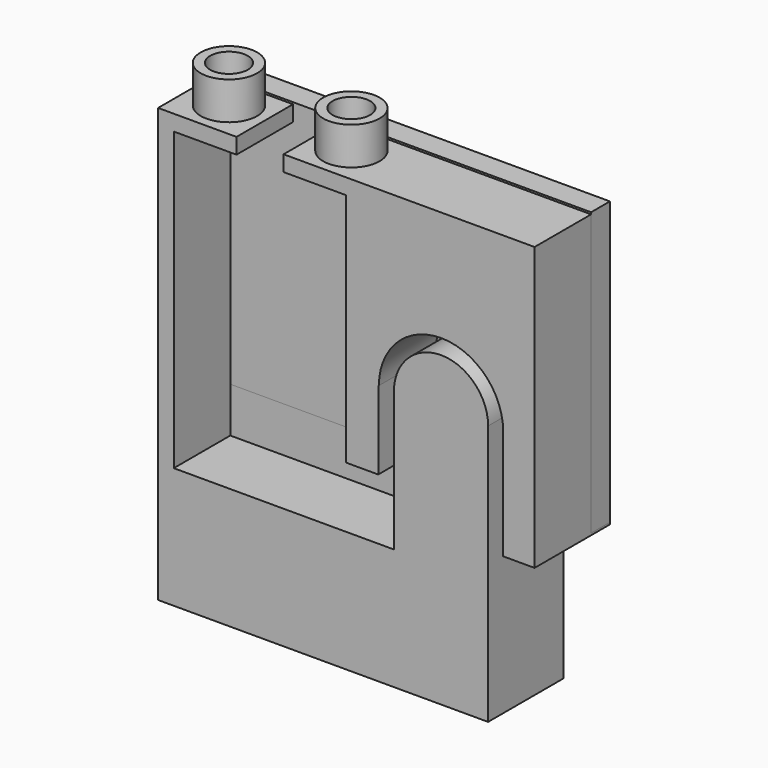
from build123d import *

# Parameters (mm, degrees)
F1_DEPTH  = 15.875
F0_W      = 2.6458333332
F0_H      = 42.3358732487
F2_W      = 63.5
F2_H      = 47.625
F2_R      = 3.175
F3_DEPTH  = 3.96875
F4_DEPTH  = 6.35
F5_R      = 4.7625
F5_R_2    = 3.175
F6_DEPTH  = 6.35
F7_R      = 3.175
F8_DEPTH  = 25.4
F9_W      = 55.6354932006
F9_H      = 15.875
F10_DEPTH = 25.4
F11_W     = 37.1146598675
F11_H     = 15.875
F12_DEPTH = 7.62
F13_W     = 37.1146598675
F13_H     = 3.96875
F14_DEPTH = 25.4


# Not quite as in the source:
# - a feature names something its author has since deleted; it is built from what else it names


with BuildPart() as f1:
    # F0 (on Front) → F1 (new body)
    with BuildSketch(Plane.XZ):
        with BuildLine():
            Line((0, 44.979166582), (-31.75, 44.979166582))
            Line((-31.75, 44.979166582), (-31.75, 42.3358732487))
            Line((-31.75, 42.3358732487), (-31.75, 2.6458333332))
            Line((-31.75, 2.6458333332), (-26.3525, 2.6458333332))
            Line((-26.3525, 2.6458333332), (-26.3525, 15.875))
            Line((-26.3525, 15.875), (-26.2466666667, 15.875))
            ThreePointArc((-26.2466666667, 15.875), (-15.7691666667, 26.3525), (-5.2916666667, 15.875))
            Line((-5.2916666667, 15.875), (-5.2916666667, 0))
            Line((-5.2916666667, 0), (0, 0))
            Line((0, 0), (0, 44.979166582))
        make_face()
        Polygon((0, -2.6458333333), (0, 0), (-5.2916666667, 0), (-5.309548229, 0), (-5.309548229, -2.6458333333), align=None)
        Polygon((-31.75, 42.3358732487), (-31.75, 44.979166582), (-34.3958333316, 44.979166582), (-37.0416664956, 44.979166582), (-42.3110765377, 44.979166582), (-42.3110765377, 42.3358732487), (-37.0416664956, 42.3358732487), (-34.3958333316, 42.3358732487), align=None)
    extrude(amount=F1_DEPTH)


with BuildPart() as f1b:
    # F0 (on Front) → F1, piece 2 (new body)
    with BuildSketch(Plane.XZ):
        with BuildLine():
            Line((-23.7066666667, 0), (-7.8316666667, 0))
            Line((-7.8316666667, 0), (-7.8316666667, 15.875))
            ThreePointArc((-7.8316666667, 15.875), (-15.7691666667, 23.8125), (-23.7066666667, 15.875))
            Line((-23.7066666667, 15.875), (-23.7066666667, 0))
        make_face()
        Polygon((-26.3525, 0), (-31.75, 0), (-60.8213265341, 0), (-63.4671598673, 0), (-63.4671598673, -2.6458333333), (-7.8316666667, -2.6458333333), (-7.8316666667, 0), (-23.7066666667, 0), align=None)
        with Locations((-62.1442432007, 21.1679366243)):
            Rectangle(F0_W, F0_H)
        Polygon((-50.2485765377, 42.3358732487), (-50.2485765377, 44.979166582), (-55.5296598693, 44.979166582), (-58.175493201, 44.979166582), (-63.4671598673, 44.979166582), (-63.4671598673, 42.3358732487), (-60.8213265341, 42.3358732487), (-58.175493201, 42.3358732487), (-55.5296598693, 42.3358732487), align=None)
    extrude(amount=F1_DEPTH)


with BuildPart() as f3:
    # F2 (on Front) → F3 (new body)
    with BuildSketch(Plane.XZ):
        with Locations((-31.75, 21.4839725468)):
            Rectangle(F2_W, F2_H)
        with Locations((-53.975, 7.1964725468)):
            Circle(F2_R, mode=Mode.SUBTRACT)
        with Locations((-9.525, 7.1964725468)):
            Circle(F2_R, mode=Mode.SUBTRACT)
        with Locations((-52.284011212, 35.7714725468)):
            Circle(F2_R, mode=Mode.SUBTRACT)
        with Locations((-9.525, 35.7714725468)):
            Circle(F2_R, mode=Mode.SUBTRACT)
        with Locations((-52.284011212, 35.7714725468)):
            Circle(F2_R)
        with Locations((-53.975, 7.1964725468)):
            Circle(F2_R)
        with Locations((-9.525, 7.1964725468)):
            Circle(F2_R)
        with Locations((-9.525, 35.7714725468)):
            Circle(F2_R)
    extrude(amount=F3_DEPTH)


with BuildPart() as f4:
    # F2 (on Front) → F4 (new body)
    with BuildSketch(Plane.XZ):
        with Locations((-9.525, 35.7714725468)):
            Circle(F2_R)
    extrude(amount=-F4_DEPTH)


with BuildPart() as f4b:
    # F2 (on Front) → F4, piece 2 (new body)
    with BuildSketch(Plane.XZ):
        with Locations((-52.284011212, 35.7714725468)):
            Circle(F2_R)
    extrude(amount=-F4_DEPTH)


with BuildPart() as f4c:
    # F2 (on Front) → F4, piece 3 (new body)
    with BuildSketch(Plane.XZ):
        with Locations((-9.525, 7.1964725468)):
            Circle(F2_R)
    extrude(amount=-F4_DEPTH)


with BuildPart() as f4d:
    # F2 (on Front) → F4, piece 4 (new body)
    with BuildSketch(Plane.XZ):
        with Locations((-53.975, 7.1964725468)):
            Circle(F2_R)
    extrude(amount=-F4_DEPTH)


with BuildPart() as f6:
    # F5 (on face) → F6 (new body)
    with BuildSketch(Plane.XY.offset(44.979166582)):
        with Locations((-56.5985765377, -9.525)):
            Circle(F5_R)
        with Locations((-56.5985765377, -9.525)):
            Circle(F5_R_2, mode=Mode.SUBTRACT)
    extrude(amount=F6_DEPTH)


with BuildPart() as f6b:
    # F5 (on face) → F6, piece 2 (new body)
    with BuildSketch(Plane.XY.offset(44.979166582)):
        with Locations((-35.9610765377, -9.525)):
            Circle(F5_R)
        with Locations((-35.9610765377, -9.525)):
            Circle(F5_R_2, mode=Mode.SUBTRACT)
    extrude(amount=F6_DEPTH)


with BuildPart() as f8_tool:
    # F7 (on face) → F8 (new body)
    with BuildSketch(Plane.XY.offset(44.979166582)):
        with Locations((-35.9610765377, -9.525)):
            Circle(F7_R)
        with Locations((-56.5985765377, -9.525)):
            Circle(F7_R)
    extrude(amount=-F8_DEPTH)


with BuildPart() as f1_1:
    add(f1.part)

    # F8: cut by f8_tool
    add(f8_tool.part, mode=Mode.SUBTRACT)


with BuildPart() as f1b_1:
    add(f1b.part)

    # F8: cut by f8_tool
    add(f8_tool.part, mode=Mode.SUBTRACT)

    # F9 (on face) → F10 (join)
    with BuildSketch(Plane(origin=(0, 0, -2.6458333333), x_dir=(1, 0, 0), z_dir=(0, 0, -1))):
        with Locations((-35.649413267, 7.9375)):
            Rectangle(F9_W, F9_H)
    extrude(amount=F10_DEPTH)


with BuildPart() as f12_tool:
    # F11 (on face) → F12 (new body)
    with BuildSketch(Plane.XY):
        with Locations((-42.2639966004, -7.9375)):
            Rectangle(F11_W, F11_H)
    extrude(amount=-F12_DEPTH)


with BuildPart() as f1b_2:
    add(f1b_1.part)

    # F12: cut by f12_tool
    add(f12_tool.part, mode=Mode.SUBTRACT)


with BuildPart() as f3_1:
    add(f3.part)

    # F12: cut by f12_tool
    add(f12_tool.part, mode=Mode.SUBTRACT)


with BuildPart() as f14:
    # F13 (on face) → F14 (new body)
    with BuildSketch(Plane(origin=(0, 0, 0), x_dir=(1, 0, 0), z_dir=(0, 0, -1))):
        with Locations((-42.2639966004, 1.984375)):
            Rectangle(F13_W, F13_H)
    extrude(amount=F14_DEPTH)


solid = Compound([f4.part, f4b.part, f4c.part, f4d.part, f6.part, f6b.part, f1_1.part, f1b_2.part, f3_1.part, f14.part])
